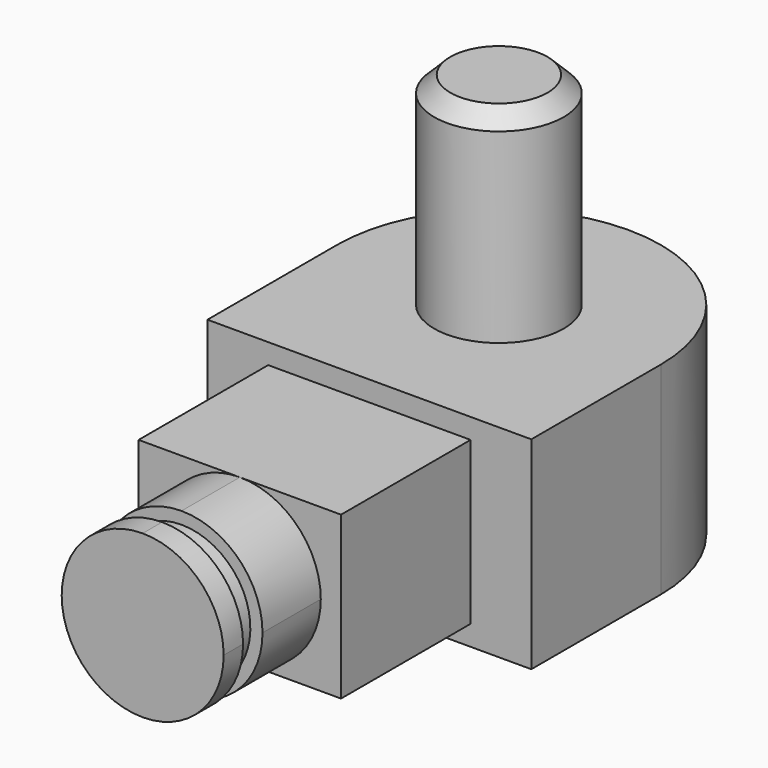
from build123d import *

# Parameters (mm, degrees)
F0_W     = 40
F0_H     = 40
F1_DEPTH = 25
F2_R     = 19.99999
F3_W     = 25
F3_H     = 20
F4_DEPTH = 20
F6_DEPTH = 15
F7_R     = 8
F8_DEPTH = 25
F9_SIZE  = 2
F10_W    = 3
F10_H    = 3


# Not quite as in the source:
# - a fillet or chamfer is up to 0.001 mm smaller than in the source, because OpenCascade refuses the exact size


with BuildPart() as f1:
    # F0 (on Top) → F1 (new body)
    with BuildSketch(Plane.XY):
        Rectangle(F0_W, F0_H)
    extrude(amount=F1_DEPTH)

    # F2 (radius 20 in the source; OpenCascade refuses exactly that, so slightly less here)
    f2_edges = [f1.edges().sort_by_distance(p)[0] for p in [
        (20, 20, 12.5),
        (-20, 20, 12.5),
    ]]
    fillet(f2_edges, radius=F2_R)

    # F3 (on face) → F4 (join)
    with BuildSketch(Plane.XZ.offset(20)):
        with Locations((0, 12.5)):
            Rectangle(F3_W, F3_H)
    extrude(amount=F4_DEPTH)

    # F5 (on face) → F6 (join)
    with BuildSketch(Plane.XZ.offset(40)):
        with BuildLine():
            ThreePointArc((0, 2.5), (7.0710678119, 5.4289321881), (10, 12.5))
            ThreePointArc((10, 12.5), (7.0710678119, 19.5710678119), (0, 22.5))
            ThreePointArc((0, 22.5), (-10, 12.5), (0, 2.5))
        make_face()
    extrude(amount=F6_DEPTH)

    # F7 (on face) → F8 (join)
    with BuildSketch(Plane.XY.offset(25)):
        Circle(F7_R)
    extrude(amount=F8_DEPTH)

    # F9
    f9_edges = [f1.edges().sort_by_distance(p)[0] for p in [
        (-8, 0, 50),
    ]]
    chamfer(f9_edges, length=F9_SIZE)

    # F10 (on Right) → F11 (revolve, cut)
    with BuildSketch(Plane.YZ):
        with Locations((-50.5, 22.5)):
            Rectangle(F10_W, F10_H)
    revolve(axis=Axis((0, -40, 12.5), (0, 1, 0)), mode=Mode.SUBTRACT)


solid = f1.part
